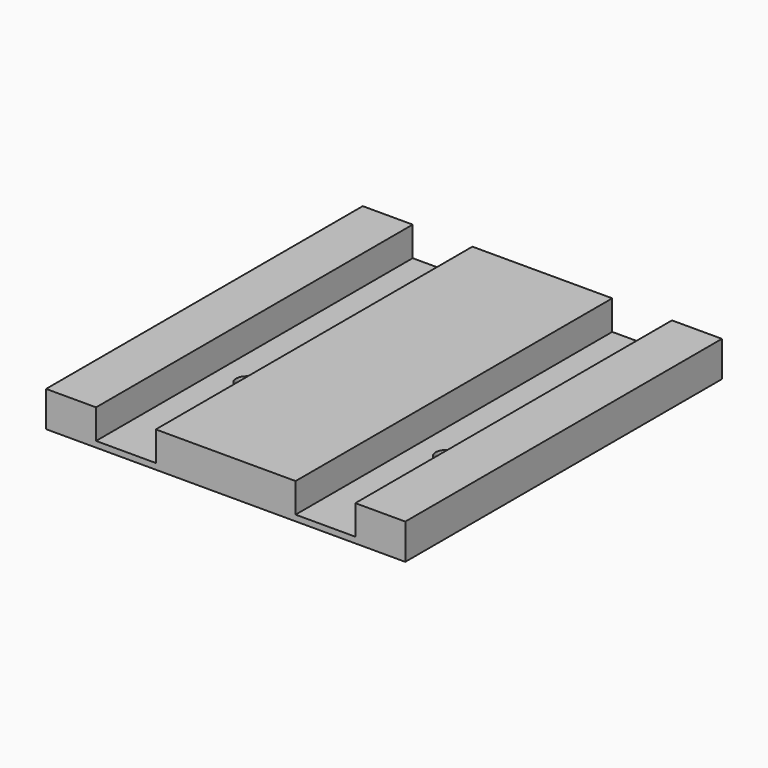
from build123d import *

# Parameters (mm, degrees)
F1_DEPTH  = 250
F2_W      = 87.5
F2_H      = 12
F3_DEPTH  = 20
F5_D      = 7
F5_DEPTH  = 40
F5_TIP    = 2.1030121666
F7_DEPTH  = 17
F8_DEPTH  = 17
F9_W      = 16.9
F9_H      = 250
F10_DEPTH = 10
F11_W     = 16.9
F11_H     = 250
F12_DEPTH = 10
F14_DEPTH = 25
F15_R     = 5
F18_W     = 250
F18_H     = 10
F19_DEPTH = 0.1
F20_W     = 250
F20_H     = 10
F21_DEPTH = 0.1
F22_W     = 143.5878481716
F22_H     = 63.6908710003
F23_DEPTH = 259


with BuildPart() as f1:
    # F0 (on Front) → F1 (new body)
    with BuildSketch(Plane.XZ):
        Polygon((-45.825098525, 2), (-45.825098525, 0), (41.674901475, 0), (41.674901475, 2), (21.674901475, 2), (21.674901475, 12), (-25.825098525, 12), (-25.825098525, 2), align=None)
    extrude(amount=F1_DEPTH)

    # F2 (on face) → F3 (join)
    with BuildSketch(Plane(origin=(0, 0, 0), x_dir=(-1, 0, 0), z_dir=(0, 1, 0))):
        with Locations((2.075098525, 6)):
            Rectangle(F2_W, F2_H)
    extrude(amount=F3_DEPTH)

    # F5
    with Locations(Plane.XY.offset(2)):
        with Locations((-35.825098525, -51), (31.674901475, -199), (31.674901475, -51), (-35.825098525, -199)):
            Hole(F5_D / 2, depth=F5_DEPTH)
            with Locations((0, 0, -(F5_DEPTH + F5_TIP / 2))):  # 118° drill point
                Cone(0, F5_D / 2, F5_TIP, mode=Mode.SUBTRACT)

    # F7 (add): a face of the model
    f7_faces = [f1.faces().sort_by_distance(p)[0] for p in [
        (-45.825098525, -125, 1.7297334649),
    ]]
    extrude(f7_faces, amount=F7_DEPTH)

    # F6 (on face) → F8 (join)
    with BuildSketch(Plane.YZ.offset(41.674901475)):
        Polygon((0, 2), (-250, 2), (-250, 0), (20, 0), (20, 12), (0, 12), align=None)
    extrude(amount=F8_DEPTH)

    # F9 (on face) → F10 (join)
    with BuildSketch(Plane.XY.offset(2)):
        with Locations((50.224901475, -125)):
            Rectangle(F9_W, F9_H)
    extrude(amount=F10_DEPTH)

    # F11 (on face) → F12 (join)
    with BuildSketch(Plane.XY.offset(2)):
        with Locations((-54.375098525, -125)):
            Rectangle(F11_W, F11_H)
    extrude(amount=F12_DEPTH)

    # F13 (on face) → F14 (cut)
    with BuildSketch(Plane.XY.offset(12)):
        with BuildLine():
            ThreePointArc((-62.825098525, 0), (-37.10740093, 13.9610044228), (-8.4745501026, 20))
            Line((-8.4745501026, 20), (-62.825098525, 20))
            Line((-62.825098525, 20), (-62.825098525, 0))
        make_face()
        with BuildLine():
            ThreePointArc((4.3243530527, 20), (32.95720388, 13.9610044228), (58.674901475, 0))
            Line((58.674901475, 0), (58.674901475, 20))
            Line((58.674901475, 20), (4.3243530527, 20))
        make_face()
    extrude(amount=-F14_DEPTH, mode=Mode.SUBTRACT)

    # F15
    f15_edges = [f1.edges().sort_by_distance(p)[0] for p in [
        (-37.107401, 13.961004, 12),
        (-2.075099, 20, 12),
        (32.957204, 13.961004, 12),
    ]]
    fillet(f15_edges, radius=F15_R)

    # F18 (on face) → F19 (cut)
    with BuildSketch(Plane.YZ.offset(21.674901475)):
        with Locations((-125, 7)):
            Rectangle(F18_W, F18_H)
    extrude(amount=-F19_DEPTH, mode=Mode.SUBTRACT)

    # F20 (on face) → F21 (cut)
    with BuildSketch(Plane(origin=(-25.825098525, 0, 0), x_dir=(0, -1, 0), z_dir=(-1, 0, 0))):
        with Locations((125, 7)):
            Rectangle(F20_W, F20_H)
    extrude(amount=-F21_DEPTH, mode=Mode.SUBTRACT)

    # F22 (on offset) → F23 (cut)
    with BuildSketch(Plane(origin=(-112.825098525, 0, 0), x_dir=(0, -1, 0), z_dir=(-1, 0, 0))):
        with Locations((44.3292455748, 5.149319768)):
            Rectangle(F22_W, F22_H)
    extrude(amount=-F23_DEPTH, mode=Mode.SUBTRACT)


solid = f1.part
